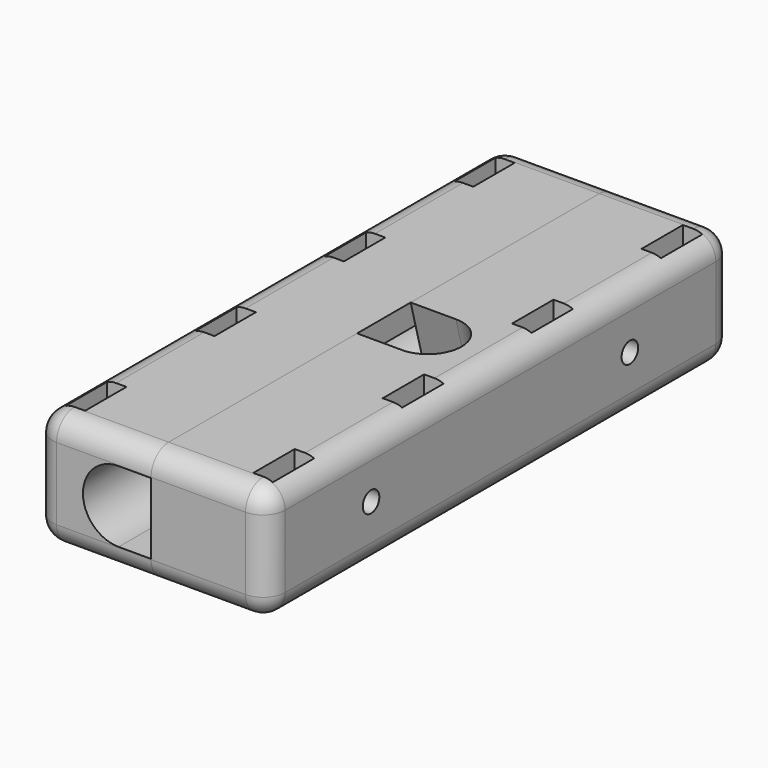
from build123d import *

# Parameters (mm, degrees)
F0_W         = 18
F0_H         = 90
F0_W_2       = 3
F0_H_2       = 8
F1_DEPTH     = 18
F3_T1_DEPTH  = 23.1
F3_T3_DEPTH  = 83.2
F3_T5_DEPTH  = 11.2
F3_S9_W      = 3.4
F3_S9_H      = 3.4
F3_T10_DEPTH = 3.4
F3_S15_W     = 3.4
F3_S15_H     = 3.4
F3_T16_DEPTH = 3.4
F3_S21_W     = 3.4
F3_S21_H     = 3.4
F3_T22_DEPTH = 3.4
F3_S27_W     = 3.4
F3_S27_H     = 3.4
F3_T28_DEPTH = 3.4
F5_DEPTH     = 90.001
F7_DEPTH     = 12
F8_R         = 4.99999
F9_R         = 1.6
F10_DEPTH    = 18.001


# Not quite as in the source:
# - a fillet or chamfer that OpenCascade refuses, or shapes differently, is made with other operations: its cross-section is extruded or revolved along the edge and cut away or added
# - a fillet or chamfer is up to 0.001 mm smaller than in the source, because OpenCascade refuses the exact size


with BuildPart() as f1:
    # F0 (on Top) → F1 (new body)
    with BuildSketch(Plane.XY):
        with Locations((10.0719179884, 38.8917037249)):
            Rectangle(F0_W, F0_H)
        with Locations((4.5719179884, 1.3917037249)):
            Rectangle(F0_W_2, F0_H_2, mode=Mode.SUBTRACT)
        with Locations((4.5719179884, 26.3917037249)):
            Rectangle(F0_W_2, F0_H_2, mode=Mode.SUBTRACT)
        with Locations((4.5719179884, 51.3917037249)):
            Rectangle(F0_W_2, F0_H_2, mode=Mode.SUBTRACT)
        with Locations((4.5719179884, 76.3917037249)):
            Rectangle(F0_W_2, F0_H_2, mode=Mode.SUBTRACT)
    extrude(amount=F1_DEPTH)

    # F3: fillet of radius 3.4 on 8 edges, made by hand

    # F3_s2 → F3_t1 (cut)
    with BuildSketch(Plane.YZ.offset(4.4719179884)):
        with BuildLine():
            ThreePointArc((-6.1082962751, 14.6), (-5.1124593312, 17.004163056), (-2.7082962751, 18))
            Line((-2.7082962751, 18), (-6.1082962751, 18))
            Line((-6.1082962751, 18), (-6.1082962751, 14.6))
        make_face()
        with BuildLine():
            ThreePointArc((-6.1082962751, 3.4), (-5.1124593312, 0.995836944), (-2.7082962751, 0))
            Line((-2.7082962751, 0), (-6.1082962751, 0))
            Line((-6.1082962751, 0), (-6.1082962751, 3.4))
        make_face()
        with BuildLine():
            ThreePointArc((83.8917037249, 14.6), (82.8958667809, 17.004163056), (80.4917037249, 18))
            Line((80.4917037249, 18), (83.8917037249, 18))
            Line((83.8917037249, 18), (83.8917037249, 14.6))
        make_face()
        with BuildLine():
            ThreePointArc((83.8917037249, 3.4), (82.8958667809, 0.995836944), (80.4917037249, 0))
            Line((80.4917037249, 0), (83.8917037249, 0))
            Line((83.8917037249, 0), (83.8917037249, 3.4))
        make_face()
    extrude(amount=F3_T1_DEPTH, mode=Mode.SUBTRACT)

    # F3_s4 → F3_t3 (cut)
    with BuildSketch(Plane.XZ.offset(-80.4917037249)):
        with BuildLine():
            ThreePointArc((1.0719179884, 14.6), (2.0677549323, 17.004163056), (4.4719179884, 18))
            Line((4.4719179884, 18), (1.0719179884, 18))
            Line((1.0719179884, 18), (1.0719179884, 14.6))
        make_face()
        with BuildLine():
            ThreePointArc((1.0719179884, 3.4), (2.0677549323, 0.995836944), (4.4719179884, 0))
            Line((4.4719179884, 0), (1.0719179884, 0))
            Line((1.0719179884, 0), (1.0719179884, 3.4))
        make_face()
    extrude(amount=F3_T3_DEPTH, mode=Mode.SUBTRACT)

    # F3_s6 → F3_t5 (cut)
    with BuildSketch(Plane.XY.offset(3.4)):
        with BuildLine():
            ThreePointArc((1.0719179884, -2.7082962751), (2.0677549323, -5.1124593312), (4.4719179884, -6.1082962751))
            Line((4.4719179884, -6.1082962751), (1.0719179884, -6.1082962751))
            Line((1.0719179884, -6.1082962751), (1.0719179884, -2.7082962751))
        make_face()
        with BuildLine():
            ThreePointArc((4.4719179884, 83.8917037249), (2.0677549323, 82.8958667809), (1.0719179884, 80.4917037249))
            Line((1.0719179884, 80.4917037249), (1.0719179884, 83.8917037249))
            Line((1.0719179884, 83.8917037249), (4.4719179884, 83.8917037249))
        make_face()
    extrude(amount=F3_T5_DEPTH, mode=Mode.SUBTRACT)


with BuildPart() as f3_tool8:
    # F3_s9 → F3_t10 (new body)
    with BuildSketch(Plane.YZ.offset(4.4719179884)):
        with Locations((-4.4082962751, 16.3)):
            Rectangle(F3_S9_W, F3_S9_H)
    extrude(amount=-F3_T10_DEPTH)

    # F3_s11 → F3_t12 (revolve, cut)
    with BuildSketch(Plane(origin=(4.4719179884, -2.7082962751, 14.6), x_dir=(0, 0.7071067812, -0.7071067812), z_dir=(0, 0.7071067812, 0.7071067812))):
        with BuildLine():
            ThreePointArc((0, -3.4), (3.4, 0), (0, 3.4))
            Line((0, 3.4), (0, -3.4))
        make_face()
    revolve(axis=Axis((4.4719179884, -2.7082962751, 14.6), (-1, 0, 0)), mode=Mode.SUBTRACT)


with BuildPart() as f1_1:
    add(f1.part)

    # F3_t7: cut F3_tool8
    add(f3_tool8.part, mode=Mode.SUBTRACT)


with BuildPart() as f3_tool14:
    # F3_s15 → F3_t16 (new body)
    with BuildSketch(Plane.XZ.offset(-80.4917037249)):
        with Locations((2.7719179884, 16.3)):
            Rectangle(F3_S15_W, F3_S15_H)
    extrude(amount=-F3_T16_DEPTH)

    # F3_s17 → F3_t18 (revolve, cut)
    with BuildSketch(Plane(origin=(4.4719179884, 80.4917037249, 14.6), x_dir=(0.7071067812, 0, -0.7071067812), z_dir=(0.7071067812, 0, 0.7071067812))):
        with BuildLine():
            ThreePointArc((0, -3.4), (3.4, 0), (0, 3.4))
            Line((0, 3.4), (0, -3.4))
        make_face()
    revolve(axis=Axis((4.4719179884, 80.4917037249, 14.6), (0, 1, 0)), mode=Mode.SUBTRACT)


with BuildPart() as f1_2:
    add(f1_1.part)

    # F3_t13: cut F3_tool14
    add(f3_tool14.part, mode=Mode.SUBTRACT)


with BuildPart() as f3_tool20:
    # F3_s21 → F3_t22 (new body)
    with BuildSketch(Plane.YZ.offset(4.4719179884)):
        with Locations((-4.4082962751, 1.7)):
            Rectangle(F3_S21_W, F3_S21_H)
    extrude(amount=-F3_T22_DEPTH)

    # F3_s23 → F3_t24 (revolve, cut)
    with BuildSketch(Plane(origin=(4.4719179884, -2.7082962751, 3.4), x_dir=(0, 0.7071067812, 0.7071067812), z_dir=(0, -0.7071067812, 0.7071067812))):
        with BuildLine():
            ThreePointArc((0, -3.4), (3.4, 0), (0, 3.4))
            Line((0, 3.4), (0, -3.4))
        make_face()
    revolve(axis=Axis((4.4719179884, -2.7082962751, 3.4), (-1, 0, 0)), mode=Mode.SUBTRACT)


with BuildPart() as f1_3:
    add(f1_2.part)

    # F3_t19: cut F3_tool20
    add(f3_tool20.part, mode=Mode.SUBTRACT)


with BuildPart() as f3_tool26:
    # F3_s27 → F3_t28 (new body)
    with BuildSketch(Plane.XZ.offset(-80.4917037249)):
        with Locations((2.7719179884, 1.7)):
            Rectangle(F3_S27_W, F3_S27_H)
    extrude(amount=-F3_T28_DEPTH)

    # F3_s29 → F3_t30 (revolve, cut)
    with BuildSketch(Plane(origin=(4.4719179884, 80.4917037249, 3.4), x_dir=(0.7071067812, 0, 0.7071067812), z_dir=(-0.7071067812, 0, 0.7071067812))):
        with BuildLine():
            ThreePointArc((0, -3.4), (3.4, 0), (0, 3.4))
            Line((0, 3.4), (0, -3.4))
        make_face()
    revolve(axis=Axis((4.4719179884, 80.4917037249, 3.4), (0, 1, 0)), mode=Mode.SUBTRACT)


with BuildPart() as f1_4:
    add(f1_3.part)

    # F3_t25: cut F3_tool26
    add(f3_tool26.part, mode=Mode.SUBTRACT)


with BuildPart() as f4_1:
    # F4: instance of F1
    add(f1_4.part.mirror(Plane(origin=(19.0719179884, 38.8917037249, 9), x_dir=(0, 1, 0), z_dir=(1, 0, 0))))

    # F6 (on face) → F7 (cut)
    with BuildSketch(Plane(origin=(19.0719179884, 0, 0), x_dir=(0, -1, 0), z_dir=(-1, 0, 0))):
        Polygon((-39.876718396, -5.0858661007), (-32.9742111659, 20.6746415815), (-42.6334694288, 23.2628320326), (-49.5359766589, -2.4976756497), align=None)
    extrude(amount=-F7_DEPTH, mode=Mode.SUBTRACT)

    # F8 (radius 5 in the source; OpenCascade refuses exactly that, so slightly less here)
    f8_edges = [f4_1.edges().sort_by_distance(p)[0] for p in [
        (31.071918, 46.455184, 9),
        (31.071918, 36.102422, 9),
    ]]
    fillet(f8_edges, radius=F8_R)

    # F9 (on face) → F10 (cut, through all)
    with BuildSketch(Plane(origin=(19.0719179884, 0, 0), x_dir=(0, -1, 0), z_dir=(-1, 0, 0))):
        with Locations((-63.8917037249, 9)):
            Circle(F9_R)
        with Locations((-13.8917037249, 9)):
            Circle(F9_R)
    extrude(amount=-F10_DEPTH, mode=Mode.SUBTRACT)


with BuildPart() as f1_5:
    add(f1_4.part)

    # F2 (on face) → F5 (cut, through all)
    with BuildSketch(Plane.XZ.offset(6.1082962751)):
        with BuildLine():
            Line((19.0719179884, 6.7612328898), (19.0719179884, 11.2387671102))
            ThreePointArc((19.0719179884, 11.2387671102), (17.042909252, 13.613199492), (14.0481821448, 14.5))
            Line((14.0481821448, 14.5), (14.0481821448, 3.5))
            ThreePointArc((14.0481821448, 3.5), (17.042909252, 4.386800508), (19.0719179884, 6.7612328898))
        make_face()
        with BuildLine():
            ThreePointArc((14.0481821448, 14.5), (17.042909252, 13.613199492), (19.0719179884, 11.2387671102))
            Line((19.0719179884, 11.2387671102), (19.0719179884, 14.5))
            Line((19.0719179884, 14.5), (14.0481821448, 14.5))
        make_face()
        with BuildLine():
            Line((14.0481821448, 3.5), (14.0481821448, 14.5))
            ThreePointArc((14.0481821448, 14.5), (8.5481821448, 9), (14.0481821448, 3.5))
        make_face()
        with BuildLine():
            Line((19.0719179884, 3.5), (19.0719179884, 6.7612328898))
            ThreePointArc((19.0719179884, 6.7612328898), (17.042909252, 4.386800508), (14.0481821448, 3.5))
            Line((14.0481821448, 3.5), (19.0719179884, 3.5))
        make_face()
    extrude(amount=-F5_DEPTH, mode=Mode.SUBTRACT)


solid = Compound([f4_1.part, f1_5.part])
